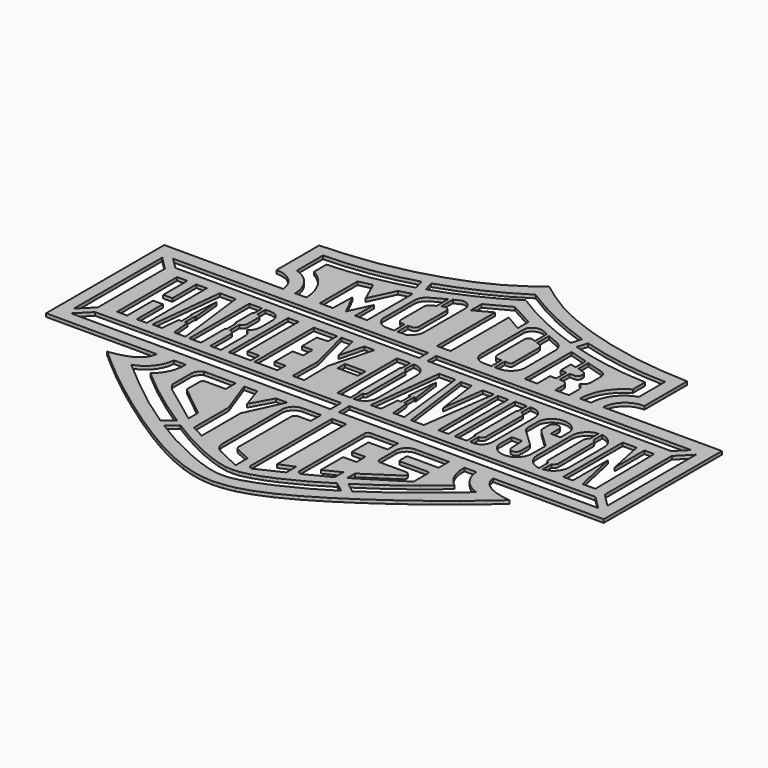
from build123d import *

# Parameters (mm, degrees)
F0_W     = 19.6540374
F0_H     = 9.0600276
F1_DEPTH = 3.175
F3_DEPTH = 3.175


# Not quite as in the source:
# - ends of sketch curves that miss each other by under 0.0002 mm in the source are joined


with BuildPart() as f1:
    # F0 (on Top) → F1 (new body)
    with BuildSketch(Plane.XY):
        with BuildLine():
            Line((14.1420596, 193.0371044), (2.54e-05, 203.2))
            Line((2.54e-05, 203.2), (-14.1420088, 193.0371044))
            Line((-14.1420088, 193.0371044), (-29.859478, 183.1781706))
            Line((-29.859478, 183.1781706), (-48.6996994, 173.9280748))
            Line((-48.6996994, 173.9280748), (-70.8524618, 165.6306822))
            Line((-70.8524618, 165.6306822), (-94.5721502, 158.685738))
            Line((-94.5721502, 158.685738), (-124.8544874, 152.3056898))
            Line((-124.8544874, 152.3056898), (-152.1199904, 149.0714824))
            Line((-152.1199904, 149.0714824), (-177.6405388, 147.5119986))
            Line((-177.6405388, 147.5119986), (-177.6405388, 95.9255638))
            ThreePointArc((-177.6405388, 95.9255638), (-161.8126826937, 90.2401239386), (-154.5155565557, 75.0876583695))
            Line((-154.5155565557, 75.0876583695), (-269.2283668, 75.0876578))
            Line((-269.2283668, 75.0876578), (-269.2283668, -67.591813))
            Line((-269.2283668, -67.591813), (-162.4395278, -67.591813))
            Line((-162.4395278, -67.591813), (-163.660328, -72.7300552))
            Line((-163.660328, -72.7300552), (-166.824914, -77.614653))
            Line((-166.824914, -77.614653), (-172.8248766, -81.9361074))
            Line((-172.8248766, -81.9361074), (-178.8491216, -84.5120992))
            Line((-178.8491216, -84.5120992), (-185.7224632, -86.3016562))
            Line((-185.7224632, -86.3016562), (-190.4166118, -87.1250226))
            Line((-190.4166118, -87.1250226), (-193.5474666, -87.557229))
            Line((-193.5474666, -87.557229), (-194.1966906, -87.6419126))
            Line((-194.1966906, -87.6419126), (-194.2412168, -87.650447))
            Line((-194.2412168, -87.650447), (-194.2444172, -87.6518186))
            Line((-194.2444172, -87.6518186), (-181.1110424, -99.1400862))
            Line((-181.1110424, -99.1400862), (-166.2656314, -111.6313236))
            Line((-166.2656314, -111.6313236), (-148.881084, -125.454156))
            Line((-148.881084, -125.454156), (-128.5152624, -140.6715246))
            Line((-128.5152624, -140.6715246), (-106.2984412, -156.2636194))
            Line((-106.2984412, -156.2636194), (-85.7835978, -169.672889))
            Line((-85.7835978, -169.672889), (-66.1549604, -181.3471608))
            Line((-66.1549604, -181.3471608), (-48.4638858, -190.4240286))
            Line((-48.4638858, -190.4240286), (-33.0758038, -196.8118238))
            Line((-33.0758038, -196.8118238), (-20.0657968, -200.7450646))
            Line((-20.0657968, -200.7450646), (-9.3675454, -202.5553734))
            Line((-9.3675454, -202.5553734), (2.54e-05, -203.2))
            Line((2.54e-05, -203.2), (9.3675708, -202.5553734))
            Line((9.3675708, -202.5553734), (20.0658222, -200.7450646))
            Line((20.0658222, -200.7450646), (33.0758292, -196.8118238))
            Line((33.0758292, -196.8118238), (48.4639112, -190.4240286))
            Line((48.4639112, -190.4240286), (66.1549858, -181.3471608))
            Line((66.1549858, -181.3471608), (85.7836232, -169.672889))
            Line((85.7836232, -169.672889), (106.2984666, -156.2636194))
            Line((106.2984666, -156.2636194), (128.5152878, -140.6715246))
            Line((128.5152878, -140.6715246), (148.8811094, -125.454156))
            Line((148.8811094, -125.454156), (166.2656822, -111.6313236))
            Line((166.2656822, -111.6313236), (181.1110932, -99.1400862))
            Line((181.1110932, -99.1400862), (194.2448236, -87.6521996))
            Line((194.2448236, -87.6521996), (194.244341, -87.6515138))
            Line((194.244341, -87.6515138), (194.2412422, -87.650447))
            Line((194.2412422, -87.650447), (194.196716, -87.6419126))
            Line((194.196716, -87.6419126), (193.547492, -87.557229))
            Line((193.547492, -87.557229), (190.4166372, -87.1250226))
            Line((190.4166372, -87.1250226), (185.722514, -86.3016562))
            Line((185.722514, -86.3016562), (178.8491724, -84.5120992))
            Line((178.8491724, -84.5120992), (172.8249274, -81.9361074))
            Line((172.8249274, -81.9361074), (166.8249394, -77.614653))
            Line((166.8249394, -77.614653), (163.6603788, -72.7300552))
            Line((163.6603788, -72.7300552), (162.4395532, -67.591813))
            Line((162.4395532, -67.591813), (269.2283922, -67.591813))
            Line((269.2283922, -67.591813), (269.2283922, 75.0876578))
            Line((269.2283922, 75.0876578), (154.5156168, 75.0876578))
            ThreePointArc((154.5156168, 75.0876578), (161.8127240681, 90.2401154451), (177.6405642737, 95.9255654857))
            Line((177.6405642737, 95.9255654857), (177.6405642, 147.5119986))
            Line((177.6405642, 147.5119986), (152.1200412, 149.0714824))
            Line((152.1200412, 149.0714824), (124.8545128, 152.3056898))
            Line((124.8545128, 152.3056898), (94.5721756, 158.685738))
            Line((94.5721756, 158.685738), (70.8525126, 165.6306822))
            Line((70.8525126, 165.6306822), (48.6997248, 173.9280748))
            Line((48.6997248, 173.9280748), (29.8595034, 183.1781706))
            Line((29.8595034, 183.1781706), (14.1420596, 193.0371044))
        make_face()
        Polygon((-65.6113496, -143.6995856), (-65.6113496, -101.8163826), (-78.06309, -67.6306496), (-65.384934, -67.6306496), (-58.36666, -88.459056), (-47.0468706, -67.8570398), (-36.179887, -67.8570398), (-52.706778, -103.4011648), (-52.706778, -150.491444), align=None, mode=Mode.SUBTRACT)
        with BuildLine():
            ThreePointArc((-32.3212796016, -79.3701489899), (-29.2933774435, -71.253843565), (-21.3300056, -67.8439588))
            Line((-21.3300056, -67.8439588), (-3.5304222, -67.8439588))
            Line((-3.5304222, -67.8439588), (-3.5304222, -80.210406))
            Line((-3.5304222, -80.210406), (-15.2329642, -80.210406))
            ThreePointArc((-15.2329642, -80.210406), (-18.1497615752, -81.3529906456), (-19.5144147135, -84.1727297137))
            Line((-19.5144147135, -84.1727297137), (-19.5144136, -145.3255412))
            ThreePointArc((-19.5144136, -145.3255412), (-19.2296744212, -148.6895309929), (-16.8327317593, -151.0669557986))
            Line((-16.8327317593, -151.0669557986), (-2.6136346, -157.5672236))
            Line((-2.6136346, -157.5672236), (-2.6136346, -172.1876922))
            Line((-2.6136346, -172.1876922), (-25.5635506, -161.3471246))
            ThreePointArc((-25.5635506, -161.3471246), (-30.4663735526, -157.0313023964), (-32.321301513, -150.768456435))
            Line((-32.321301513, -150.768456435), (-32.3212796016, -79.3701489899))
        make_face(mode=Mode.SUBTRACT)
        with BuildLine():
            ThreePointArc((-122.3827372, -76.2915416), (-120.8287362555, -71.0640079916), (-116.6714450023, -67.5342833566))
            Line((-116.6714450023, -67.5342833566), (-86.2076254, -67.534282))
            Line((-86.2076254, -67.534282), (-86.2076254, -79.547593))
            Line((-86.2076254, -79.547593), (-105.6910764, -79.547593))
            ThreePointArc((-105.6910764, -79.547593), (-107.9361404303, -80.4775289697), (-108.8660764, -82.722593))
            Line((-108.8660764, -82.722593), (-108.8660764, -96.8522066))
            ThreePointArc((-108.8660764, -96.8522066), (-108.5538044409, -98.2253100789), (-107.6784145645, -99.3283148407))
            Line((-107.6784145645, -99.3283148407), (-78.06309, -123.0975694))
            Line((-78.06309, -123.0975694), (-78.06309, -134.643749))
            Line((-78.06309, -134.643749), (-115.909979, -106.5612296))
            ThreePointArc((-115.909979, -106.5612296), (-119.7249141769, -102.820046366), (-122.3827159776, -98.1847176848))
            Line((-122.3827159776, -98.1847176848), (-122.3827372, -76.2915416))
        make_face(mode=Mode.SUBTRACT)
        with BuildLine():
            Line((-145.996279, -67.3619176), (-134.717536, -67.3619176))
            ThreePointArc((-134.717536, -67.3619176), (-137.310340691, -82.5887413046), (-146.7862264728, -94.7865420589))
            Line((-146.7862264728, -94.7865420589), (-127.245237, -111.1028512))
            Line((-127.245237, -111.1028512), (-104.9677606, -127.7255256))
            Line((-104.9677606, -127.7255256), (-79.2877256, -145.0411374))
            Line((-79.2877256, -145.0411374), (-56.846851, -158.4920122))
            Line((-56.846851, -158.4920122), (-35.6108, -169.163873))
            Line((-35.6108, -169.163873), (-24.9636026, -173.5323428))
            Line((-24.9636026, -173.5323428), (-15.6519118, -176.6936776))
            Line((-15.6519118, -176.6936776), (-6.2742318, -178.9238992))
            Line((-6.2742318, -178.9238992), (2.54e-05, -179.1750544))
            Line((2.54e-05, -179.1750544), (6.2742826, -178.9238992))
            Line((6.2742826, -178.9238992), (15.6519626, -176.6936776))
            Line((15.6519626, -176.6936776), (24.963628, -173.5323428))
            Line((24.963628, -173.5323428), (35.6108254, -169.163873))
            Line((35.6108254, -169.163873), (56.8468764, -158.4920122))
            Line((56.8468764, -158.4920122), (79.287751, -145.0411374))
            Line((79.287751, -145.0411374), (104.967786, -127.7255256))
            Line((104.967786, -127.7255256), (127.2452624, -111.1028512))
            Line((127.2452624, -111.1028512), (146.7862444, -94.7865516))
            ThreePointArc((146.7862444, -94.7865516), (137.310366091, -82.5887413046), (134.7175669292, -67.3619180279))
            Line((134.7175669292, -67.3619180279), (145.9963044, -67.3619176))
            ThreePointArc((145.9963044, -67.3619176), (152.3423659864, -83.4100130014), (166.6724387901, -93.0257694748))
            Line((166.6724387901, -93.0257694748), (142.6379926, -113.3297962))
            Line((142.6379926, -113.3297962), (117.1181808, -133.4640968))
            Line((117.1181808, -133.4640968), (89.2798824, -152.7536188))
            Line((89.2798824, -152.7536188), (64.9414754, -167.274494))
            Line((64.9414754, -167.274494), (40.9417266, -179.20716))
            Line((40.9417266, -179.20716), (26.8981682, -184.9550276))
            Line((26.8981682, -184.9550276), (14.9882352, -188.8931706))
            Line((14.9882352, -188.8931706), (6.1493908, -190.747777))
            Line((6.1493908, -190.747777), (2.54e-05, -190.961391))
            Line((2.54e-05, -190.961391), (-6.1493654, -190.747777))
            Line((-6.1493654, -190.747777), (-14.9881844, -188.8931706))
            Line((-14.9881844, -188.8931706), (-26.8981174, -184.9550276))
            Line((-26.8981174, -184.9550276), (-40.9417012, -179.20716))
            Line((-40.9417012, -179.20716), (-64.94145, -167.274494))
            Line((-64.94145, -167.274494), (-89.279857, -152.7536188))
            Line((-89.279857, -152.7536188), (-117.11813, -133.4640968))
            Line((-117.11813, -133.4640968), (-142.6379418, -113.3297962))
            Line((-142.6379418, -113.3297962), (-166.6724124, -93.0257728))
            ThreePointArc((-166.6724124, -93.0257728), (-152.3423405864, -83.4100130014), (-145.996279, -67.3619176))
        make_face(mode=Mode.SUBTRACT)
        with BuildLine():
            Line((6.7564762, -165.5422394), (6.7564762, -67.4467028))
            Line((6.7564762, -67.4467028), (20.6506572, -67.4467028))
            Line((20.6506572, -67.4467028), (20.6506572, -151.2936776))
            Line((20.6506572, -151.2936776), (34.5582748, -145.4559194))
            Line((34.5582748, -145.4559194), (34.5582748, -157.3994566))
            Line((34.5582748, -157.3994566), (11.2897158, -168.4120584))
            ThreePointArc((11.2897158, -168.4120584), (8.2332086772, -168.2248710223), (6.7564762, -165.5422394))
        make_face(mode=Mode.SUBTRACT)
        with BuildLine():
            ThreePointArc((40.952928, -70.8255124), (41.8828639697, -68.5804483697), (44.127928, -67.6505124))
            Line((44.127928, -67.6505124), (70.695312, -67.6505124))
            Line((70.695312, -67.6505124), (70.695312, -80.357853))
            Line((70.695312, -80.357853), (52.2235684, -80.357853))
            Line((52.2235684, -80.357853), (52.2235684, -100.280978))
            Line((52.2235684, -100.280978), (65.281302, -100.280978))
            Line((65.281302, -100.280978), (65.281302, -111.0502224))
            Line((65.281302, -111.0502224), (52.3817342, -111.0502224))
            Line((52.3817342, -111.0502224), (52.3817342, -137.8996734))
            Line((52.3817342, -137.8996734), (67.9736004, -130.3002474))
            Line((67.9736004, -130.3002474), (67.9736004, -140.6656572))
            Line((67.9736004, -140.6656572), (45.5774552, -152.1580396))
            ThreePointArc((45.5774552, -152.1580396), (42.4728817254, -152.0427652409), (40.952928, -149.3332548))
            Line((40.952928, -149.3332548), (40.952928, -70.8255124))
        make_face(mode=Mode.SUBTRACT)
        with BuildLine():
            ThreePointArc((76.5355594, -77.8897858), (79.6601442583, -70.3463706583), (87.2035594, -67.2217858))
            Line((87.2035594, -67.2217858), (119.4482752, -67.2217858))
            Line((119.4482752, -67.2217858), (119.4482752, -79.7066986))
            Line((119.4482752, -79.7066986), (90.621485, -79.7066986))
            ThreePointArc((90.621485, -79.7066986), (89.4989529849, -80.1716665849), (89.033985, -81.2941986))
            Line((89.033985, -81.2941986), (89.033985, -88.2090946))
            ThreePointArc((89.033985, -88.2090946), (89.4989529849, -89.3316266151), (90.621485, -89.7965946))
            Line((90.621485, -89.7965946), (117.3354016, -89.7965946))
            ThreePointArc((117.3354016, -89.7965946), (118.4579336151, -90.2615625849), (118.9229016, -91.3840946))
            Line((118.9229016, -91.3840946), (118.9229016, -108.3329304))
            ThreePointArc((118.9229016, -108.3329304), (118.7231270904, -109.103887087), (118.1740836936, -109.6808059862))
            Line((118.1740836936, -109.6808059862), (76.0884686, -135.867394))
            Line((76.0884686, -135.867394), (76.0884686, -126.5390154))
            Line((76.0884686, -126.5390154), (106.6129948, -106.2993556))
            ThreePointArc((106.6129948, -106.2993556), (107.8983541652, -102.7369444158), (104.858439, -100.478209))
            Line((104.858439, -100.478209), (79.7105594, -100.478209))
            ThreePointArc((79.7105594, -100.478209), (77.4654953697, -99.5482730303), (76.5355594, -97.303209))
            Line((76.5355594, -97.303209), (76.5355594, -77.8897858))
        make_face(mode=Mode.SUBTRACT)
        Polygon((241.5389124, -42.9606964), (254.4726432, -55.8944272), (-254.4726178, -55.8944272), (-241.538887, -42.9606964), align=None, mode=Mode.SUBTRACT)
        Polygon((-257.6546536, 58.1261474), (-244.7209228, 45.1924166), (-244.7209228, -35.6750874), (-257.6546536, -48.6088182), align=None, mode=Mode.SUBTRACT)
        Polygon((-228.9712718, 40.27424), (-219.072968, 40.27424), (-219.072968, 11.1252762), (-210.2015608, 11.1252762), (-210.2015608, 40.0207734), (-200.0757746, 40.0207734), (-200.0757746, -32.4714616), (-209.7076324, -32.4714616), (-209.7076324, -1.041273), (-219.0859728, -1.041273), (-219.0859728, -32.217995), (-228.9712718, -32.217995), align=None, mode=Mode.SUBTRACT)
        Polygon((-172.1001384, 39.878254), (-163.326064, -31.7719202), (-174.3281502, -31.7719202), (-176.1367064, -13.5614664), (-178.409727, -13.5614664), (-178.409727, -1.399032), (-177.5347986, -1.399032), (-180.3527762, 27.133169), (-182.4662848, -1.399032), (-181.584727, -1.399032), (-181.584727, -13.5614664), (-184.1844932, -13.5614664), (-186.064271, -31.8222884), (-195.1947074, -31.8222884), (-187.4069912, 39.878254), align=None, mode=Mode.SUBTRACT)
        Polygon((-159.3887592, -32.1777614), (-159.3887592, 40.3503638), (-146.8873872, 40.3503638), (-146.8873872, 30.2785526), (-148.0862672, 30.2785526), (-148.0862672, 9.0406982), (-146.8873872, 9.0406982), (-146.8873872, -2.7298904), (-148.0302856, -2.7298904), (-148.0302856, -32.1777614), align=None, mode=Mode.SUBTRACT)
        with BuildLine():
            Line((-139.7143256, 14.0983462), (-139.7143256, 26.6478258))
            ThreePointArc((-139.7143256, 26.6478258), (-140.7777408591, 29.2151373409), (-143.3450524, 30.2785526))
            Line((-143.3450524, 30.2785526), (-143.7123872, 30.2785526))
            Line((-143.7123872, 30.2785526), (-143.7123872, 40.3503638))
            Line((-143.7123872, 40.3503638), (-138.630914, 40.3503638))
            ThreePointArc((-138.630914, 40.3503638), (-131.5177339488, 37.4039934117), (-128.5713456, 30.2908208))
            Line((-128.5713456, 30.2908208), (-128.5713456, 15.621127))
            ThreePointArc((-128.5713456, 15.621127), (-129.8878680564, 10.0153075785), (-133.5621706253, 5.581579644))
            ThreePointArc((-133.5621706253, 5.581579644), (-130.5434654932, 2.410157842), (-128.8906905592, -1.6443179244))
            Line((-128.8906905592, -1.6443179244), (-128.8906998, -31.9702434))
            Line((-128.8906998, -31.9702434), (-139.1825258, -31.9702434))
            Line((-139.1825258, -31.9702434), (-139.1825258, -7.0280022))
            ThreePointArc((-139.1825258, -7.0280022), (-140.4414135999, -3.9887781999), (-143.4806376, -2.7298904))
            Line((-143.4806376, -2.7298904), (-143.7123872, -2.7298904))
            Line((-143.7123872, -2.7298904), (-143.7123872, 9.0406982))
            Line((-143.7123872, 9.0406982), (-143.236696, 9.0406982))
            ThreePointArc((-143.236696, 9.0406982), (-140.6816922783, 11.016674021), (-139.7143256, 14.0983462))
        make_face(mode=Mode.SUBTRACT)
        Polygon((-111.852202, 40.3556724), (-111.8080314, -21.1233004), (-100.6105938, -21.1233004), (-100.6105938, -31.2598308), (-121.869835, -31.2598308), (-121.869835, 40.3556724), align=None, mode=Mode.SUBTRACT)
        Polygon((-74.6178594, 40.2731732), (-74.6178594, 29.42463), (-85.0053672, 28.9729926), (-85.0053672, 11.127867), (-74.8436654, 11.127867), (-74.8436654, -0.1719326), (-85.2311732, -0.1719326), (-85.2311732, -21.6255854), (-74.8333276, -21.6255854), (-74.8333276, -31.316041), (-96.9735932, -31.316041), (-96.9735932, 40.2731732), align=None, mode=Mode.SUBTRACT)
        Polygon((-59.8341958, 40.3967188), (-54.098825, 16.3799266), (-48.0050094, 40.038274), (-38.319964, 40.038274), (-49.4330482, -1.54305), (-49.0746288, -31.2952384), (-60.1926406, -31.2952384), (-59.8341958, -1.54305), (-70.5879716, 40.3967188), align=None, mode=Mode.SUBTRACT)
        with Locations((-31.6882907, 4.1863772)):
            Rectangle(F0_W, F0_H, mode=Mode.SUBTRACT)
        Polygon((-16.5874954, -31.8487044), (-16.5874954, 40.3389338), (-4.036187, 40.3389338), (-4.036187, 29.384625), (-4.8898302, 29.384625), (-4.8898302, -20.7723994), (-4.036187, -20.7723994), (-4.036187, -31.8487044), align=None, mode=Mode.SUBTRACT)
        Polygon((-84.6643214, 97.608644), (-94.4688484, 75.8681998), (-105.125901, 97.1823558), (-105.765346, 74.1630724), (-118.3406828, 74.1630724), (-118.3406828, 119.7753256), (-105.5522146, 122.5461862), (-96.3871326, 102.0845812), (-84.8774782, 126.5958606), (-73.1546924, 129.7930094), (-73.1546924, 74.802492), (-84.6643214, 74.802492), align=None, mode=Mode.SUBTRACT)
        with BuildLine():
            ThreePointArc((-65.6251929538, 122.4955132045), (-63.8885401272, 128.5718081325), (-59.3120744507, 132.9299367451))
            Line((-59.3120744507, 132.9299367451), (-46.780704, 139.6986792))
            Line((-46.780704, 139.6986792), (-46.780704, 125.6666524))
            Line((-46.780704, 125.6666524), (-50.0226076, 124.1410522))
            ThreePointArc((-50.0226076, 124.1410522), (-52.7265302483, 121.696264216), (-53.6112566596, 118.1599612954))
            Line((-53.6112566596, 118.1599612954), (-53.6112466, 91.843225))
            ThreePointArc((-53.6112466, 91.843225), (-52.1245261385, 88.3742006081), (-48.5871522783, 87.0583533015))
            Line((-48.5871522783, 87.0583533015), (-46.780704, 87.0583476))
            Line((-46.780704, 87.0583476), (-46.780704, 74.459211))
            Line((-46.780704, 74.459211), (-53.6856178, 74.459211))
            ThreePointArc((-53.6856178, 74.459211), (-61.3544163414, 77.1659174561), (-65.6251871908, 84.0867011733))
            Line((-65.6251871908, 84.0867011733), (-65.6251929538, 122.4955132045))
        make_face(mode=Mode.SUBTRACT)
        with BuildLine():
            ThreePointArc((-27.2517879875, 87.0646213745), (-29.2583487026, 79.6635449929), (-34.9981082212, 74.5785299309))
            Line((-34.9981082212, 74.5785299309), (-43.605704, 74.459211))
            Line((-43.605704, 74.459211), (-43.605704, 87.0583476))
            Line((-43.605704, 87.0583476), (-40.6921208, 87.0583476))
            ThreePointArc((-40.6921208, 87.0583476), (-37.5288637552, 87.9149030186), (-36.146486, 90.8862546))
            Line((-36.146486, 90.8862546), (-36.1465114, 123.901835))
            ThreePointArc((-36.1465114, 123.901835), (-37.9658265527, 127.4199998167), (-41.8883312279, 127.968951887))
            Line((-41.8883312279, 127.968951887), (-43.605704, 127.160782))
            Line((-43.605704, 127.160782), (-43.605704, 141.413611))
            Line((-43.605704, 141.413611), (-36.8284506, 144.551146))
            ThreePointArc((-36.8284506, 144.551146), (-30.0949481247, 142.1330206236), (-27.251787, 135.567674))
            Line((-27.251787, 135.567674), (-27.2517879875, 87.0646213745))
        make_face(mode=Mode.SUBTRACT)
        with BuildLine():
            ThreePointArc((0.7791703001, 40.3389315779), (9.0704763175, 36.5724206665), (12.460732, 28.1202892))
            Line((12.460732, 28.1202892), (12.460732, -19.7829424))
            ThreePointArc((12.460732, -19.7829424), (8.9267521304, -28.3147245304), (0.39497, -31.8487044))
            Line((0.39497, -31.8487044), (-0.861187, -31.8487044))
            Line((-0.861187, -31.8487044), (-0.861187, -20.7723994))
            ThreePointArc((-0.861187, -20.7723994), (0.9875603671, -20.0066231671), (1.7533366, -18.1578758))
            Line((1.7533366, -18.1578758), (1.7533112, 26.7701014))
            ThreePointArc((1.7533112, 26.7701014), (0.9875439474, 28.6188397869), (-0.861187, 29.3846249999))
            Line((-0.861187, 29.3846249999), (-0.861187, 40.3389338))
            Line((-0.861187, 40.3389338), (0.7791703001, 40.3389315779))
        make_face(mode=Mode.SUBTRACT)
        Polygon((39.5045438, 40.4753572), (47.606585, -31.3533536), (36.949507, -31.3533536), (35.2861626, -13.2645404), (33.0837286, -13.2645404), (33.0837286, -1.4310868), (34.9180658, -1.4310868), (30.9185818, 27.6298914), (28.2041092, -1.4310868), (29.9087286, -1.4310868), (29.9087286, -13.2645404), (26.680287, -13.2645404), (25.2240542, -31.7796164), (15.632684, -31.7796164), (23.945215, 40.4753572), align=None, mode=Mode.SUBTRACT)
        Polygon((55.3894244, 40.26154), (61.1247698, -1.3198094), (66.5016704, 39.9030698), (77.2614152, 39.9030698), (67.2185854, -32.1473322), (54.672484, -32.1473322), (44.994068, 40.26154), align=None, mode=Mode.SUBTRACT)
        Polygon((90.9559268, 39.9893536), (90.6873726, -31.979743), (81.0198786, -31.979743), (81.0198786, 39.9893536), align=None, mode=Mode.SUBTRACT)
        Polygon((97.0040986, 40.6366726), (108.4756276, 40.6366726), (108.4756276, 29.4205152), (107.3417716, 29.4205152), (107.3417716, -21.5382856), (108.4756276, -21.5382856), (108.4756276, -31.9697354), (97.0040986, -31.9697354), align=None, mode=Mode.SUBTRACT)
        with BuildLine():
            ThreePointArc((114.0653294, 40.6366726), (121.8095954093, 37.4289083698), (125.0173776, 29.6846498))
            Line((125.0173776, 29.6846498), (125.0173776, -21.4315548))
            ThreePointArc((125.0173776, -21.4315548), (121.9308159636, -28.8831737636), (114.479197, -31.9697354))
            Line((114.479197, -31.9697354), (111.6506276, -31.9697354))
            Line((111.6506276, -31.9697354), (111.6506276, -21.5382856))
            Line((111.6506276, -21.5382856), (111.6946204, -21.5382856))
            ThreePointArc((111.6946204, -21.5382856), (114.5294358103, -20.3640666103), (115.7036548, -17.5292512))
            Line((115.7036548, -17.5292512), (115.7036548, 25.4398018))
            ThreePointArc((115.7036548, 25.4398018), (114.5377382786, 28.2545732786), (111.7229668, 29.4204898))
            Line((111.7229668, 29.4204898), (111.7229668, 40.6369012))
            Line((111.7229668, 40.6369012), (114.0653294, 40.6366726))
        make_face(mode=Mode.SUBTRACT)
        Polygon((-250.1738456, 61.8667038), (250.1738964, 61.8667038), (239.4611162, 51.1539236), (-239.4610654, 51.1539236), align=None, mode=Mode.SUBTRACT)
        with BuildLine():
            ThreePointArc((105.629456, 101.9267202), (108.1623932811, 102.9508805937), (109.2716602404, 105.4477191137))
            Line((109.2716602404, 105.4477191137), (109.2716636, 107.2017922))
            ThreePointArc((109.2716636, 107.2017922), (108.4671286209, 109.5322179519), (106.3962303909, 110.8699553098))
            Line((106.3962303909, 110.8699553098), (100.7466616, 112.2591862))
            Line((100.7466616, 112.2591862), (100.7466616, 124.3797614))
            Line((100.7466616, 124.3797614), (117.0134566, 119.61876))
            ThreePointArc((117.0134566, 119.61876), (120.7858974955, 117.003149826), (122.2365348, 112.6478824))
            Line((122.2365348, 112.6478824), (122.2365348, 100.9953784))
            ThreePointArc((122.2365348, 100.9953784), (120.7341211216, 96.475317793), (116.8247802009, 93.7540592023))
            ThreePointArc((116.8247802009, 93.7540592023), (120.7770726041, 90.07130742), (122.2365348, 84.870036))
            Line((122.2365348, 84.870036), (122.2365348, 74.2273344))
            Line((122.2365348, 74.2273344), (108.9898506, 74.2273344))
            Line((108.9898506, 74.2273344), (108.9898506, 84.1953358))
            ThreePointArc((108.9898506, 84.1953358), (107.3964700923, 88.0421093318), (103.549704, 89.6355077999))
            Line((103.549704, 89.6355077999), (100.7466616, 89.6355078))
            Line((100.7466616, 89.6355078), (100.7466616, 101.9267202))
            Line((100.7466616, 101.9267202), (105.629456, 101.9267202))
        make_face(mode=Mode.SUBTRACT)
        with BuildLine():
            ThreePointArc((131.0061388, 27.7267924), (145.2482573223, 39.2003381401), (160.1894537018, 28.6532606966))
            Line((160.1894537018, 28.6532606966), (160.1894434, 16.4942266))
            Line((160.1894434, 16.4942266), (150.7647734, 16.4942266))
            Line((150.7647734, 16.4942266), (150.7647734, 25.864439))
            ThreePointArc((150.7647734, 25.864439), (145.9258059269, 30.7658650831), (141.0243798439, 25.92689761))
            Line((141.0243798439, 25.92689761), (141.0541756, 19.5079366))
            ThreePointArc((141.0541756, 19.5079366), (141.568756434, 17.003863287), (143.029099429, 14.9056319058))
            Line((143.029099429, 14.9056319058), (159.3387212, -0.598551))
            ThreePointArc((159.3387212, -0.598551), (160.0688887318, -1.6476733363), (160.3261715999, -2.8997148))
            Line((160.3261715999, -2.8997148), (160.0972455914, -18.1098948808))
            ThreePointArc((160.0972455914, -18.1098948808), (147.4401925639, -32.5061107429), (131.2267124, -22.2799148))
            Line((131.2267124, -22.2799148), (131.2267124, -6.1261244))
            Line((131.2267124, -6.1261244), (141.3714724, -6.1261244))
            Line((141.3714724, -6.1261244), (142.1043386, -19.9026018))
            ThreePointArc((142.1043386, -19.9026018), (146.3764927145, -23.8469185362), (150.4331002, -19.6812408))
            Line((150.4331002, -19.6812408), (150.4331002, -10.53846))
            ThreePointArc((150.4331002, -10.53846), (150.073733135, -8.2979480295), (148.949555738, -6.3268407881))
            Line((148.949555738, -6.3268407881), (132.9930440044, 8.7631181005))
            ThreePointArc((132.9930440044, 8.7631181005), (131.5239800251, 10.8651253753), (131.0061388, 13.376783))
            Line((131.0061388, 13.376783), (131.0061388, 27.7267924))
        make_face(mode=Mode.SUBTRACT)
        with BuildLine():
            ThreePointArc((164.9569472, 23.7957614), (168.9626334878, 34.1868039394), (178.9066799387, 39.2003084894))
            Line((178.9066799387, 39.2003084894), (178.906678, 28.4255718))
            ThreePointArc((178.906678, 28.4255718), (177.0951399085, 26.8214836492), (176.2841264378, 24.5417849404))
            Line((176.2841264378, 24.5417849404), (176.284128, -18.9544706))
            ThreePointArc((176.284128, -18.9544706), (177.2569518927, -20.7871387597), (178.9066807595, -22.0454922775))
            Line((178.9066807595, -22.0454922775), (178.906678, -32.6573896))
            ThreePointArc((178.906678, -32.6573896), (168.9781517056, -27.8362436107), (164.9569472, -17.5576738))
            Line((164.9569472, -17.5576738), (164.9569472, 23.7957614))
        make_face(mode=Mode.SUBTRACT)
        with BuildLine():
            ThreePointArc((182.3047157316, 39.2003309317), (192.068135581, 34.1523429225), (195.9867048, 23.8833914))
            Line((195.9867048, 23.8833914), (195.9867048, -19.4109848))
            ThreePointArc((195.9867048, -19.4109848), (191.4968543807, -28.462643774), (182.3047155513, -32.6573913341))
            Line((182.3047155513, -32.6573913341), (182.3047154, -22.0454982))
            ThreePointArc((182.3047154, -22.0454982), (184.5934642044, -20.5265987609), (185.6899581417, -18.0080420615))
            Line((185.6899581417, -18.0080420615), (185.250582, 24.6071898))
            ThreePointArc((185.250582, 24.6071898), (184.4175473867, 27.010059744), (182.3047124647, 28.4255610633))
            Line((182.3047124647, 28.4255610633), (182.3047157316, 39.2003309317))
        make_face(mode=Mode.SUBTRACT)
        Polygon((215.5312174, 39.200328), (222.9579488, 3.0803342), (222.9579488, 39.3491212), (232.345611, 39.3491212), (233.250613, -32.6573896), (220.8084992, -32.6573896), (211.4866738, 9.7783142), (211.4866738, -32.6573896), (202.1437918, -32.6573896), (202.1437918, 39.200328), align=None, mode=Mode.SUBTRACT)
        Polygon((244.7209482, -35.6750874), (244.7209482, 45.1924166), (257.654679, 58.1261474), (257.654679, -48.6088182), align=None, mode=Mode.SUBTRACT)
        Polygon((0.361696, 161.315146), (23.6936026, 148.5905842), (23.6936026, 135.4859876), (7.4948288, 145.0380386), (7.4948288, 74.7406938), (-5.7422034, 74.7406938), (-5.7422034, 145.0380386), (-22.0946472, 136.296654), (-22.0946472, 149.3334072), align=None, mode=Mode.SUBTRACT)
        with BuildLine():
            ThreePointArc((39.1472166, 74.768075), (31.6597664144, 77.8694784144), (28.558363, 85.3569286))
            Line((28.558363, 85.3569286), (28.558363, 138.1711994))
            ThreePointArc((28.558363, 138.1711994), (33.6934567233, 144.0245647106), (41.4793980216, 144.1259090255))
            Line((41.4793980216, 144.1259090255), (46.8830406, 141.8041868))
            Line((46.8830406, 141.8041868), (46.8830406, 127.221488))
            Line((46.8830406, 127.221488), (44.0848496, 128.2802616))
            ThreePointArc((44.0848496, 128.2802616), (40.6174581315, 127.7676515829), (39.0154668, 124.6500936))
            Line((39.0154668, 124.6500936), (39.0154668, 91.7134056))
            ThreePointArc((39.0154668, 91.7134056), (40.4075883862, 88.3525267862), (43.7684672, 86.9604052))
            Line((43.7684672, 86.9604052), (46.8830406, 86.9603798))
            Line((46.8830406, 86.9603798), (46.8830406, 74.768075))
            Line((46.8830406, 74.768075), (39.1472166, 74.768075))
        make_face(mode=Mode.SUBTRACT)
        with BuildLine():
            Line((56.2555644, 88.9874014), (56.2555644, 119.5638198))
            ThreePointArc((56.2555644, 119.5638198), (55.512832916, 122.5008344949), (53.4632137608, 124.7317012982))
            Line((53.4632137608, 124.7317012982), (50.0580406, 126.0201442))
            Line((50.0580406, 126.0201442), (50.0580406, 140.4400036))
            Line((50.0580406, 140.4400036), (61.1239316, 135.6854538))
            ThreePointArc((61.1239316, 135.6854538), (66.5233646269, 131.1646758344), (68.5454814, 124.4191314))
            Line((68.5454814, 124.4191314), (68.5454814, 86.3708204))
            ThreePointArc((68.5454814, 86.3708204), (63.4007430429, 78.0302558356), (54.1599882, 74.768075))
            Line((54.1599882, 74.768075), (50.0580406, 74.768075))
            Line((50.0580406, 74.768075), (50.0580406, 86.9603798))
            Line((50.0580406, 86.9603798), (54.2285428, 86.9603798))
            ThreePointArc((54.2285428, 86.9603798), (55.661863519, 87.554080681), (56.2555644, 88.9874014))
        make_face(mode=Mode.SUBTRACT)
        with BuildLine():
            ThreePointArc((-165.1474724219, 136.5513279217), (-79.0450488117, 149.992283986), (1.97826e-05, 186.682388679))
            ThreePointArc((1.97826e-05, 186.682388679), (79.0450844137, 149.9922808891), (165.1474978219, 136.5513279217))
            Line((165.1474978219, 136.5513279217), (165.147498, 104.9371536))
            ThreePointArc((165.147498, 104.9371536), (149.1278838278, 93.7117917706), (143.017582697, 75.1295170408))
            Line((143.017582697, 75.1295170408), (132.178425, 75.129517))
            ThreePointArc((132.178425, 75.129517), (138.1196358993, 96.3230696513), (153.8567368198, 111.7116454731))
            Line((153.8567368198, 111.7116454731), (153.8567408, 126.615444))
            ThreePointArc((153.8567408, 126.615444), (73.6885284593, 140.4625783295), (2.91039e-05, 174.9399657669))
            ThreePointArc((2.91039e-05, 174.9399657669), (-73.688474209, 140.462587391), (-153.8566904153, 126.6154549979))
            Line((-153.8566904153, 126.6154549979), (-153.85669, 111.7116384))
            ThreePointArc((-153.85669, 111.7116384), (-138.1196048569, 96.3230601296), (-132.178403967, 75.129516949))
            Line((-132.178403967, 75.129516949), (-143.0175194, 75.129517))
            ThreePointArc((-143.0175194, 75.129517), (-149.1278402816, 93.711801541), (-165.1474721979, 104.9371549461))
            Line((-165.1474721979, 104.9371549461), (-165.1474724219, 136.5513279217))
        make_face(mode=Mode.SUBTRACT)
        Polygon((79.551149, 74.1344212), (79.551149, 130.5832796), (97.5716616, 125.3090204), (97.5716616, 113.0399314), (91.9534864, 114.4214374), (91.9534864, 101.9267202), (97.5716616, 101.9267202), (97.5716616, 89.6355078), (91.5936446, 89.6355078), (91.5936446, 74.1344212), align=None, mode=Mode.SUBTRACT)
    extrude(amount=F1_DEPTH)

    # F2 (on face) → F3 (join)
    with BuildSketch(Plane.XY.offset(3.175)):
        with BuildLine():
            ThreePointArc((3.9751254, 61.8667038), (2.54e-05, 65.8418038), (-3.9750746, 61.8667038))
            Line((-3.9750746, 61.8667038), (-3.9750746, 51.1539236))
            ThreePointArc((-3.9750746, 51.1539236), (2.54e-05, 47.1788236), (3.9751254, 51.1539236))
            Line((3.9751254, 51.1539236), (3.9751254, 61.8667038))
        make_face()
        with BuildLine():
            ThreePointArc((3.9751127, -42.9606964), (1.27e-05, -38.9855964), (-3.9750873, -42.9606964))
            Line((-3.9750873, -42.9606964), (-3.9750873, -55.8944272))
            ThreePointArc((-3.9750873, -55.8944272), (1.27e-05, -59.8695272), (3.9751127, -55.8944272))
            Line((3.9751127, -55.8944272), (3.9751127, -42.9606964))
        make_face()
        with BuildLine():
            ThreePointArc((86.8510354805, -155.9003826379), (92.4266462379, -155.1824657195), (91.7087293195, -149.6068549621))
            Line((91.7087293195, -149.6068549621), (81.7165979195, -141.8943735621))
            ThreePointArc((81.7165979195, -141.8943735621), (76.1409871621, -142.6122904805), (76.8589040805, -148.1879012379))
            Line((76.8589040805, -148.1879012379), (86.8510354805, -155.9003826379))
        make_face()
        with BuildLine():
            ThreePointArc((-91.7086785195, -149.6068549621), (-92.4265954379, -155.1824657195), (-86.8509846805, -155.9003826379))
            Line((-86.8509846805, -155.9003826379), (-76.8588532805, -148.1879012379))
            ThreePointArc((-76.8588532805, -148.1879012379), (-76.1409363621, -142.6122904805), (-81.7165471195, -141.8943735621))
            Line((-81.7165471195, -141.8943735621), (-91.7086785195, -149.6068549621))
        make_face()
        with BuildLine():
            ThreePointArc((80.5869140536, 149.537553267), (77.9331415792, 154.4933914074), (72.9773034388, 151.839618933))
            Line((72.9773034388, 151.839618933), (69.8837231519, 141.6136111625))
            ThreePointArc((69.8837231519, 141.6136111625), (72.5374956263, 136.6577730221), (77.4933337668, 139.3115454965))
            Line((77.4933337668, 139.3115454965), (80.5869140536, 149.537553267))
        make_face()
        with BuildLine():
            ThreePointArc((-72.9772526388, 151.839618933), (-77.9330907792, 154.4933914074), (-80.5868632536, 149.537553267))
            Line((-80.5868632536, 149.537553267), (-77.4932829668, 139.3115454965))
            ThreePointArc((-77.4932829668, 139.3115454965), (-72.5374448263, 136.6577730221), (-69.8836723519, 141.6136111625))
            Line((-69.8836723519, 141.6136111625), (-72.9772526388, 151.839618933))
        make_face()
    extrude(amount=-F3_DEPTH)


solid = f1.part
